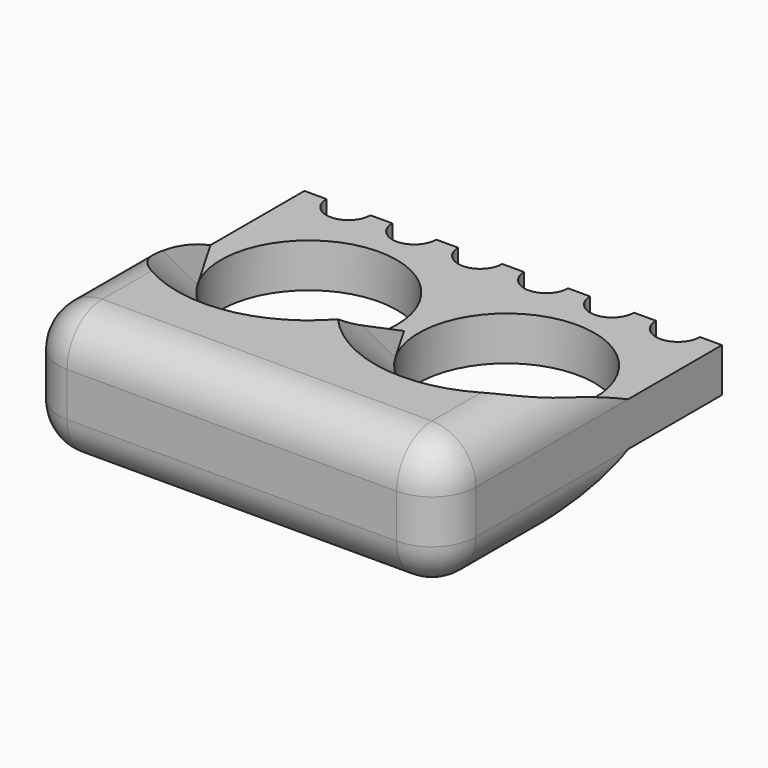
from build123d import *

# Parameters (mm, degrees)
F0_R           = 12.7
F1_DEPTH       = 6.35
F3_START       = 6.35
F3_DEPTH       = 6.35
F4_DEPTH       = 6.35
F5_T1_DEPTH    = 26.0831417175
F5_T3_DEPTH    = 22.9081417175
F5_T5_DEPTH    = 22.9081417175
F5_T7_DEPTH    = 26.0831417175
F5_T10_ANGLE   = 120
F5_T12_ANGLE   = 120
F5_2_T1_DEPTH  = 22.9081417175
F5_2_T3_DEPTH  = 26.0831417175
F5_2_T5_DEPTH  = 26.0831417175
F5_2_T7_DEPTH  = 22.9081417175
F5_2_T10_ANGLE = 120
F5_2_T12_ANGLE = 120
F6_R           = 6.34999
F6_2_R         = 6.34999


# Not quite as in the source:
# - a fillet or chamfer that OpenCascade refuses, or shapes differently, is made with other operations: its cross-section is extruded or revolved along the edge and cut away or added
# - a fillet or chamfer is up to 0.001 mm smaller than in the source, because OpenCascade refuses the exact size


with BuildPart() as f1:
    # F0 (on Top) → F1 (new body)
    with BuildSketch(Plane.XY):
        with BuildLine():
            Line((-23.8125, -25.4), (23.8125, -25.4))
            ThreePointArc((23.8125, -25.4), (28.3026280605, -23.5401280605), (30.1625, -19.05))
            Line((30.1625, -19.05), (30.1625, 25.4))
            Line((30.1625, 25.4), (26.9875, 25.4))
            ThreePointArc((26.9875, 25.4), (23.8125, 22.225), (20.6375, 25.4))
            Line((20.6375, 25.4), (17.4625, 25.4))
            ThreePointArc((17.4625, 25.4), (14.2875, 22.225), (11.1125, 25.4))
            Line((11.1125, 25.4), (7.9375, 25.4))
            ThreePointArc((7.9375, 25.4), (4.7625, 22.225), (1.5875, 25.4))
            Line((1.5875, 25.4), (-1.5875, 25.4))
            ThreePointArc((-1.5875, 25.4), (-4.7625, 22.225), (-7.9375, 25.4))
            Line((-7.9375, 25.4), (-11.1125, 25.4))
            ThreePointArc((-11.1125, 25.4), (-14.2875, 22.225), (-17.4625, 25.4))
            Line((-17.4625, 25.4), (-20.6375, 25.4))
            ThreePointArc((-20.6375, 25.4), (-23.8125, 22.225), (-26.9875, 25.4))
            Line((-26.9875, 25.4), (-30.1625, 25.4))
            Line((-30.1625, 25.4), (-30.1625, -19.05))
            ThreePointArc((-30.1625, -19.05), (-28.3026280605, -23.5401280605), (-23.8125, -25.4))
        make_face()
        with Locations((-14.2875, 6.35)):
            Circle(F0_R, mode=Mode.SUBTRACT)
        with Locations((14.2875, 6.35)):
            Circle(F0_R, mode=Mode.SUBTRACT)
    extrude(amount=F1_DEPTH)


with BuildPart() as f3:
    # F2 (on Top) → F3 (new body)
    with BuildSketch(Plane.XY.offset(F3_START)):
        with BuildLine():
            Line((-23.8125, -25.4), (23.8125, -25.4))
            ThreePointArc((23.8125, -25.4), (28.3026280605, -23.5401280605), (30.1625, -19.05))
            Line((30.1625, -19.05), (30.1625, 0))
            Line((30.1625, 0), (30.1625, 8.4463065702))
            Line((30.1625, 8.4463065702), (25.2860226281, 0))
            ThreePointArc((25.2860226281, 0), (14.2875, -6.35), (3.2889773719, 0))
            Line((3.2889773719, 0), (0, 5.6966759131))
            Line((0, 5.6966759131), (-3.2889773719, 0))
            ThreePointArc((-3.2889773719, 0), (-14.2875, -6.35), (-25.2860226281, 0))
            Line((-25.2860226281, 0), (-30.1625, 8.4463065702))
            Line((-30.1625, 8.4463065702), (-30.1625, 0))
            Line((-30.1625, 0), (-30.1625, -19.05))
            ThreePointArc((-30.1625, -19.05), (-28.3026280605, -23.5401280605), (-23.8125, -25.4))
        make_face()
    extrude(amount=F3_DEPTH)

    # F5: chamfer of 6.35 on 2 edges, made by hand

    # F5_s2 → F5_t1 (cut)
    with BuildSketch(Plane(origin=(19.3630765157, 33.5378323161, 0), x_dir=(0, 0, 1), z_dir=(-0.5, -0.8660254038, 0))):
        Polygon((12.7, -28.2483379566), (6.35, -21.8983379566), (12.7, -21.8983379566), align=None)
    extrude(amount=F5_T1_DEPTH, mode=Mode.SUBTRACT)

    # F5_s4 → F5_t3 (cut)
    with BuildSketch(Plane(origin=(0.822244343, -1.4241689783, 0), x_dir=(0, 0, 1), z_dir=(-0.5, 0.8660254038, 0))):
        Polygon((12.7, -3.5016620434), (6.35, 2.8483379566), (12.7, 2.8483379566), align=None)
    extrude(amount=F5_T3_DEPTH, mode=Mode.SUBTRACT)

    # F5_s6 → F5_t5 (cut)
    with BuildSketch(Plane(origin=(10.6318265157, 18.4148637025, 0), x_dir=(0, 0, 1), z_dir=(-0.5, -0.8660254038, 0))):
        Polygon((12.7, -3.5016620434), (6.35, 2.8483379566), (12.7, 2.8483379566), align=None)
    extrude(amount=F5_T5_DEPTH, mode=Mode.SUBTRACT)

    # F5_s8 → F5_t7 (cut)
    with BuildSketch(Plane(origin=(-6.321505657, 10.9491689783, 0), x_dir=(0, 0, 1), z_dir=(-0.5, 0.8660254038, 0))):
        Polygon((12.7, -28.2483379566), (6.35, -21.8983379566), (12.7, -21.8983379566), align=None)
    extrude(amount=F5_T7_DEPTH, mode=Mode.SUBTRACT)

    # F5_s9 → F5_t10 (revolve, cut)
    with BuildSketch(Plane(origin=(-0.822244343, -1.4241689783, 0), x_dir=(0, 0, 1), z_dir=(0.5, 0.8660254038, 0))):
        Polygon((12.7, 3.5016620434), (6.35, -2.8483379566), (12.7, -2.8483379566), align=None)
    revolve(axis=Axis((-14.2875, 6.35, 12.7), (0, 0, -1)), revolution_arc=F5_T10_ANGLE, mode=Mode.SUBTRACT)

    # F5_s11 → F5_t12 (revolve, cut)
    with BuildSketch(Plane(origin=(6.321505657, 10.9491689783, 0), x_dir=(0, 0, 1), z_dir=(0.5, 0.8660254038, 0))):
        Polygon((12.7, 28.2483379566), (6.35, 21.8983379566), (12.7, 21.8983379566), align=None)
    revolve(axis=Axis((14.2875, 6.35, 12.7), (0, 0, -1)), revolution_arc=F5_T12_ANGLE, mode=Mode.SUBTRACT)

    # F6 (radius 6.35 in the source; OpenCascade refuses exactly that, so slightly less here)
    f6_edges = [f3.edges().sort_by_distance(p)[0] for p in [
        (0, -25.4, 12.7),
        (-28.302628, -23.540128, 12.7),
        (-30.1625, -11.615142, 12.7),
        (28.302628, -23.540128, 12.7),
        (30.1625, -11.615142, 12.7),
    ]]
    fillet(f6_edges, radius=F6_R)


with BuildPart() as f4:
    # F2 (on Top) → F4 (new body)
    with BuildSketch(Plane.XY):
        with BuildLine():
            Line((-23.8125, -25.4), (23.8125, -25.4))
            ThreePointArc((23.8125, -25.4), (28.3026280605, -23.5401280605), (30.1625, -19.05))
            Line((30.1625, -19.05), (30.1625, 0))
            Line((30.1625, 0), (30.1625, 8.4463065702))
            Line((30.1625, 8.4463065702), (25.2860226281, 0))
            ThreePointArc((25.2860226281, 0), (14.2875, -6.35), (3.2889773719, 0))
            Line((3.2889773719, 0), (0, 5.6966759131))
            Line((0, 5.6966759131), (-3.2889773719, 0))
            ThreePointArc((-3.2889773719, 0), (-14.2875, -6.35), (-25.2860226281, 0))
            Line((-25.2860226281, 0), (-30.1625, 8.4463065702))
            Line((-30.1625, 8.4463065702), (-30.1625, 0))
            Line((-30.1625, 0), (-30.1625, -19.05))
            ThreePointArc((-30.1625, -19.05), (-28.3026280605, -23.5401280605), (-23.8125, -25.4))
        make_face()
    extrude(amount=-F4_DEPTH)

    # F5#2: chamfer of 6.35 on 2 edges, made by hand

    # F5_2_s2 → F5_2_t1 (cut)
    with BuildSketch(Plane(origin=(10.6318265157, 18.4148637025, 0), x_dir=(0, 0, 1), z_dir=(-0.5, -0.8660254038, 0))):
        Polygon((-6.35, -3.5016620434), (0, 2.8483379566), (-6.35, 2.8483379566), align=None)
    extrude(amount=F5_2_T1_DEPTH, mode=Mode.SUBTRACT)

    # F5_2_s4 → F5_2_t3 (cut)
    with BuildSketch(Plane(origin=(-6.321505657, 10.9491689783, 0), x_dir=(0, 0, 1), z_dir=(-0.5, 0.8660254038, 0))):
        Polygon((-6.35, -28.2483379566), (0, -21.8983379566), (-6.35, -21.8983379566), align=None)
    extrude(amount=F5_2_T3_DEPTH, mode=Mode.SUBTRACT)

    # F5_2_s6 → F5_2_t5 (cut)
    with BuildSketch(Plane(origin=(19.3630765157, 33.5378323161, 0), x_dir=(0, 0, 1), z_dir=(-0.5, -0.8660254038, 0))):
        Polygon((-6.35, -28.2483379566), (0, -21.8983379566), (-6.35, -21.8983379566), align=None)
    extrude(amount=F5_2_T5_DEPTH, mode=Mode.SUBTRACT)

    # F5_2_s8 → F5_2_t7 (cut)
    with BuildSketch(Plane(origin=(0.822244343, -1.4241689783, 0), x_dir=(0, 0, 1), z_dir=(-0.5, 0.8660254038, 0))):
        Polygon((-6.35, -3.5016620434), (0, 2.8483379566), (-6.35, 2.8483379566), align=None)
    extrude(amount=F5_2_T7_DEPTH, mode=Mode.SUBTRACT)

    # F5_2_s9 → F5_2_t10 (revolve, cut)
    with BuildSketch(Plane(origin=(6.321505657, 10.9491689783, 0), x_dir=(0, 0, 1), z_dir=(0.5, 0.8660254038, 0))):
        Polygon((-6.35, 28.2483379566), (0, 21.8983379566), (-6.35, 21.8983379566), align=None)
    revolve(axis=Axis((14.2875, 6.35, -6.35), (0, 0, -1)), revolution_arc=F5_2_T10_ANGLE, mode=Mode.SUBTRACT)

    # F5_2_s11 → F5_2_t12 (revolve, cut)
    with BuildSketch(Plane(origin=(-0.822244343, -1.4241689783, 0), x_dir=(0, 0, 1), z_dir=(0.5, 0.8660254038, 0))):
        Polygon((-6.35, 3.5016620434), (0, -2.8483379566), (-6.35, -2.8483379566), align=None)
    revolve(axis=Axis((-14.2875, 6.35, -6.35), (0, 0, -1)), revolution_arc=F5_2_T12_ANGLE, mode=Mode.SUBTRACT)

    # F6#2 (radius 6.35 in the source; OpenCascade refuses exactly that, so slightly less here)
    f6_2_edges = [f4.edges().sort_by_distance(p)[0] for p in [
        (30.1625, -11.615142, -6.35),
        (28.302628, -23.540128, -6.35),
        (0, -25.4, -6.35),
        (-28.302628, -23.540128, -6.35),
        (-30.1625, -11.615142, -6.35),
    ]]
    fillet(f6_2_edges, radius=F6_2_R)


solid = Compound([f1.part, f3.part, f4.part])
